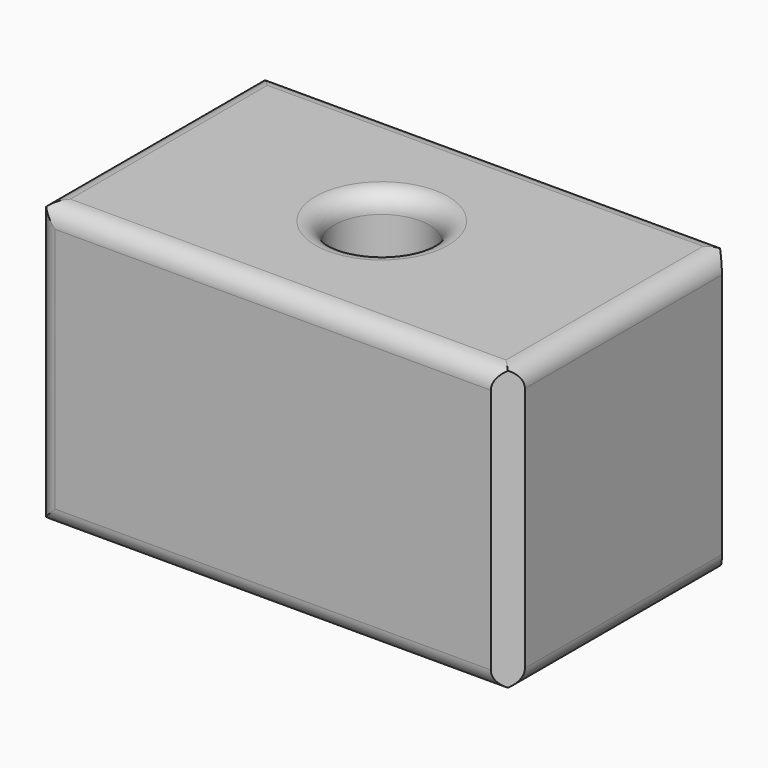
from build123d import *

# Parameters (mm, degrees)
F0_W        = 127
F0_H        = 76.2
F1_DEPTH    = 76.2
F2_R        = 12.7
F3_DEPTH    = 76.201
F4_R        = 5.08
F5_T1_DEPTH = 91.44
F6_T1_DEPTH = 92.1682991577


# Not quite as in the source:
# - a fillet or chamfer that OpenCascade refuses, or shapes differently, is made with other operations: its cross-section is extruded or revolved along the edge and cut away or added


with BuildPart() as f1:
    # F0 (on Front) → F1 (new body)
    with BuildSketch(Plane.XZ):
        with Locations((1.319276005, 11.0456193745)):
            Rectangle(F0_W, F0_H)
    extrude(amount=F1_DEPTH)

    # F2 (on face) → F3 (cut, through all)
    with BuildSketch(Plane.XY.offset(49.1456193745)):
        with Locations((0, -38.1)):
            Circle(F2_R)
    extrude(amount=-F3_DEPTH, mode=Mode.SUBTRACT)

    # F4
    f4_edges = [f1.edges().sort_by_distance(p)[0] for p in [
        (64.819276, -38.1, 49.145619),
        (1.319276, 0, 49.145619),
        (1.319276, -76.2, 49.145619),
        (-62.180724, -38.1, 49.145619),
        (-12.7, -38.1, 49.145619),
        (-62.180724, -38.1, -27.054381),
        (1.319276, 0, -27.054381),
        (1.319276, -76.2, -27.054381),
        (64.819276, -38.1, -27.054381),
        (-12.7, -38.1, -27.054381),
    ]]
    fillet(f4_edges, radius=F4_R)

    # F5: fillet of radius 5.08 on 4 edges, made by hand

    # F5_s2 → F5_t1 (cut)
    with BuildSketch(Plane.XY.offset(-34.6743806255)):
        with BuildLine():
            ThreePointArc((-57.100723995, 0), (-60.6928264434, -1.4878975516), (-62.180723995, -5.08))
            Line((-62.180723995, -5.08), (-62.180723995, 0))
            Line((-62.180723995, 0), (-57.100723995, 0))
        make_face()
        with BuildLine():
            ThreePointArc((-57.100723995, -76.2), (-60.6928264434, -74.7121024484), (-62.180723995, -71.12))
            Line((-62.180723995, -71.12), (-62.180723995, -76.2))
            Line((-62.180723995, -76.2), (-57.100723995, -76.2))
        make_face()
    extrude(amount=F5_T1_DEPTH, mode=Mode.SUBTRACT)

    # F6: chamfer of 5.08 on 4 edges, made by hand

    # F6_s2 → F6_t1 (cut)
    with BuildSketch(Plane.XY.offset(-35.0385302044)):
        Polygon((64.819276005, -5.08), (59.739276005, 0), (64.819276005, 0), align=None)
        Polygon((64.819276005, -71.12), (59.739276005, -76.2), (64.819276005, -76.2), align=None)
    extrude(amount=F6_T1_DEPTH, mode=Mode.SUBTRACT)


solid = f1.part
